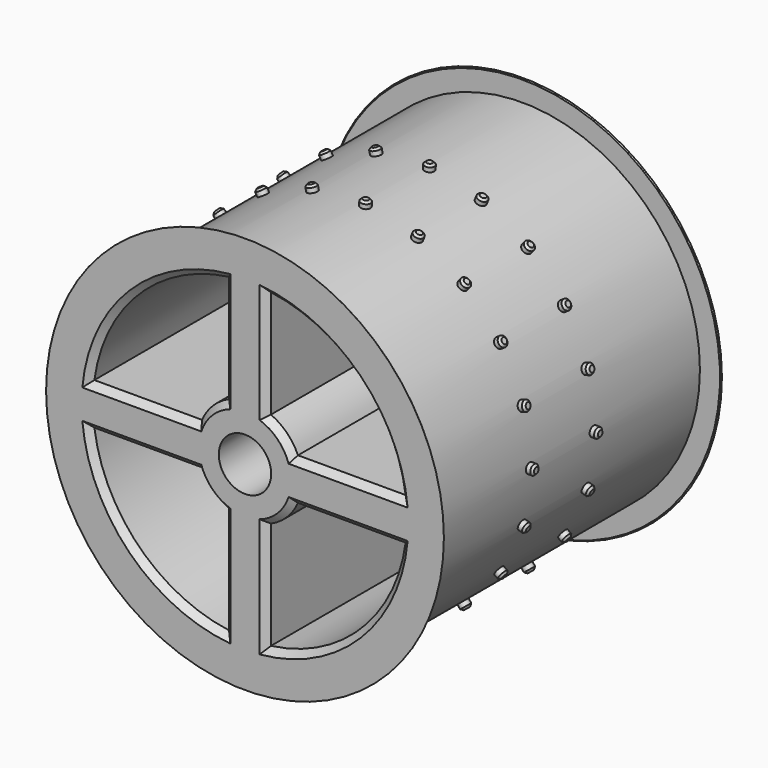
from build123d import *

# Parameters (mm, degrees)
F0_R      = 84.89324665
F1_DEPTH  = 166
F2_R      = 95
F2_R_2    = 84.89324665
F3_DEPTH  = 0.5
F4_R      = 95
F4_R_2    = 84.89324665
F5_DEPTH  = 0.5
F6_R      = 2.3876
F7_DEPTH  = 88
F8_SIZE   = 1
F9_COUNT  = 21
F9_ANGLE  = 342.8571428
F10_SIZE  = 1
F11_COUNT = 22
F11_ANGLE = 359.99999994
F12_SIZE  = 0.49999
F13_R     = 12.5
F14_DEPTH = 166.001
F15_SIZE  = 3


# Not quite as in the source:
# - a fillet or chamfer is up to 0.001 mm smaller than in the source, because OpenCascade refuses the exact size


with BuildPart() as f1:
    # F0 (on Front) → F1 (new body)
    with BuildSketch(Plane.XZ):
        Circle(F0_R)
    extrude(amount=F1_DEPTH)

    # F2 (on face) → F3 (join)
    with BuildSketch(Plane(origin=(0, 0, 0), x_dir=(-1, 0, 0), z_dir=(0, 1, 0))):
        Circle(F2_R)
        Circle(F2_R_2, mode=Mode.SUBTRACT)
    extrude(amount=-F3_DEPTH)

    # F4 (on face) → F5 (join)
    with BuildSketch(Plane.XZ.offset(166)):
        Circle(F4_R)
        Circle(F4_R_2, mode=Mode.SUBTRACT)
    extrude(amount=-F5_DEPTH)



with BuildPart() as f7:
    # F6 (on Right) → F7 (new body)
    with BuildSketch(Plane.YZ):
        with Locations((-63.95, 0)):
            Circle(F6_R)
    extrude(amount=F7_DEPTH)

    # F8
    f8_edges = [f7.edges().sort_by_distance(p)[0] for p in [
        (88, -66.3376, 0),
    ]]
    chamfer(f8_edges, length=F8_SIZE)


with BuildPart() as f7b:
    # F6 (on Right) → F7, piece 2 (new body)
    with BuildSketch(Plane.YZ):
        with Locations((-102.05, 0)):
            Circle(F6_R)
    extrude(amount=F7_DEPTH)

    # F10
    f10_edges = [f7b.edges().sort_by_distance(p)[0] for p in [
        (88, -104.4376, 0),
    ]]
    chamfer(f10_edges, length=F10_SIZE)


with BuildPart() as f1_1:
    add(f1.part)

    add(f7.part)  # F9 merges F7
    # F9: F7 ×21 about axis
    f9_axis = Axis((0, 0, 0), (0, 1, 0))
    for i in range(1, F9_COUNT):
        add(f7.part.rotate(f9_axis, i * F9_ANGLE / (F9_COUNT - 1)))


    add(f7b.part)  # F11 merges F7b
    # F11: F7b ×22 about axis
    f11_axis = Axis((0, 0, 0), (0, 1, 0))
    for i in range(1, F11_COUNT):
        add(f7b.part.rotate(f11_axis, i * F11_ANGLE / (F11_COUNT - 1)))

    # F12 (size 0.5 in the source; OpenCascade refuses exactly that, so slightly less here)
    f12_edges = [f1_1.edges().sort_by_distance(p)[0] for p in [
        (95, -0.5, 0),
        (-95, -165.5, 0),
    ]]
    chamfer(f12_edges, length=F12_SIZE)

    # F13 (on face) → F14 (cut, through all)
    with BuildSketch(Plane(origin=(0, 0, 0), x_dir=(-1, 0, 0), z_dir=(0, 1, 0))):
        with BuildLine():
            Line((-10, 22.9128784748), (-10, 74.3303437366))
            ThreePointArc((-10, 74.3303437366), (-53.033008589, 53.033008589), (-74.3303437366, 10))
            Line((-74.3303437366, 10), (-22.9128784748, 10))
            ThreePointArc((-22.9128784748, 10), (-17.6776695297, 17.6776695297), (-10, 22.9128784748))
        make_face()
        with BuildLine():
            Line((22.9128784748, 10), (74.3303437366, 10))
            ThreePointArc((74.3303437366, 10), (53.033008589, 53.033008589), (10, 74.3303437366))
            Line((10, 74.3303437366), (10, 22.9128784748))
            ThreePointArc((10, 22.9128784748), (17.6776695297, 17.6776695297), (22.9128784748, 10))
        make_face()
        with BuildLine():
            ThreePointArc((-74.3303437366, -10), (-53.033008589, -53.033008589), (-10, -74.3303437366))
            Line((-10, -74.3303437366), (-10, -22.9128784748))
            ThreePointArc((-10, -22.9128784748), (-17.6776695297, -17.6776695297), (-22.9128784748, -10))
            Line((-22.9128784748, -10), (-74.3303437366, -10))
        make_face()
        with BuildLine():
            ThreePointArc((10, -74.3303437366), (53.033008589, -53.033008589), (74.3303437366, -10))
            Line((74.3303437366, -10), (22.9128784748, -10))
            ThreePointArc((22.9128784748, -10), (17.6776695297, -17.6776695297), (10, -22.9128784748))
            Line((10, -22.9128784748), (10, -74.3303437366))
        make_face()
        Circle(F13_R)
    extrude(amount=-F14_DEPTH, mode=Mode.SUBTRACT)

    # F15
    f15_edges = [f1_1.edges().sort_by_distance(p)[0] for p in [
        (-53.033009, -166, 53.033009),
        (-10, -166, 48.621611),
        (-48.621611, -166, 10),
        (-17.67767, -166, 17.67767),
        (53.033009, -166, 53.033009),
        (48.621611, -166, 10),
        (17.67767, -166, 17.67767),
        (10, -166, 48.621611),
        (48.621611, -166, -10),
        (53.033009, -166, -53.033009),
        (17.67767, -166, -17.67767),
        (10, -166, -48.621611),
        (-10, -166, -48.621611),
        (-17.67767, -166, -17.67767),
        (-48.621611, -166, -10),
        (-53.033009, -166, -53.033009),
        (-53.033009, 0, 53.033009),
        (-10, 0, 48.621611),
        (-17.67767, 0, 17.67767),
        (-48.621611, 0, 10),
        (-53.033009, 0, -53.033009),
        (-48.621611, 0, -10),
        (-17.67767, 0, -17.67767),
        (-10, 0, -48.621611),
        (10, 0, 48.621611),
        (53.033009, 0, 53.033009),
        (17.67767, 0, 17.67767),
        (48.621611, 0, 10),
        (17.67767, 0, -17.67767),
        (10, 0, -48.621611),
        (48.621611, 0, -10),
        (53.033009, 0, -53.033009),
    ]]
    chamfer(f15_edges, length=F15_SIZE)


solid = f1_1.part
